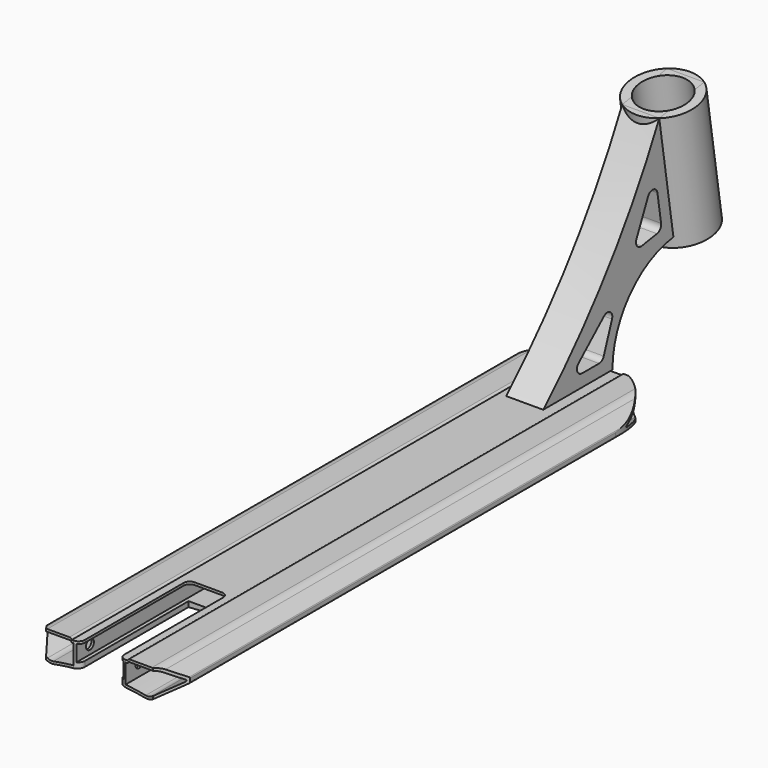
from build123d import *

# Parameters (mm, degrees)
F1_DEPTH       = 250
F2_W           = 38
F2_H           = 13
F3_DEPTH       = 250
F4_T1_DEPTH    = 509.3674969976
F5_R           = 9
F6_R           = 1
F8_DEPTH       = 500.001
F10_DEPTH      = 529
F10_DEPTH_BACK = 27.0742567341
F12_DEPTH      = 27.0742568341
F12_DEPTH_BACK = 530
F13_F1_R       = 4.9999
F13_F2_R       = 5
F13_F3_R       = 5
F13_F4_R       = 4.9999
F13_F5_R       = 5
F15_DEPTH      = 15
F16_R          = 27.5
F17_DEPTH      = 100
F19_D          = 40
F21_D          = 8
F21_DEPTH      = 66
F21_TIP        = 2.4034424761
F23_DEPTH      = 72.5010001
F24_R          = 5


# Not quite as in the source:
# - a fillet or chamfer that OpenCascade refuses, or shapes differently, is made with other operations: its cross-section is extruded or revolved along the edge and cut away or added
# - a fillet or chamfer is up to 0.001 mm smaller than in the source, because OpenCascade refuses the exact size
# - an extrude ends at something that could not be found from the text; its depth is read off the source's solid


with BuildPart() as f1:
    # F0 (on Front) → F1 (new body, symmetric)
    with BuildSketch(Plane.XZ):
        with BuildLine():
            Line((22.5, 25.7732567341), (0, 25.7732567341))
            Line((0, 25.7732567341), (-22.5, 25.7732567341))
            Line((-22.5, 25.7732567341), (-22.5, 27.0732567341))
            Line((-22.5, 27.0732567341), (-45.5824640741, 27.0732567341))
            Line((-45.5824640741, 27.0732567341), (-57.5, 17.0732567341))
            Line((-57.5, 17.0732567341), (-57.5, 13.0732567341))
            Line((-57.5, 13.0732567341), (-40.1794919243, 3.0732567341))
            ThreePointArc((-40.1794919243, 3.0732567341), (0, 7.1508015925), (40.1794919243, 3.0732567341))
            Line((40.1794919243, 3.0732567341), (57.5, 13.0732567341))
            Line((57.5, 13.0732567341), (57.5, 17.0732567341))
            Line((57.5, 17.0732567341), (45.5824640741, 27.0732567341))
            Line((45.5824640741, 27.0732567341), (22.5, 27.0732567341))
            Line((22.5, 27.0732567341), (22.5, 25.7732567341))
        make_face()
    extrude(amount=F1_DEPTH, both=True)

    # F2 (on Front) → F3 (cut, symmetric)
    with BuildSketch(Plane.XZ):
        with Locations((0, 17.2732567341)):
            Rectangle(F2_W, F2_H)
    extrude(amount=F3_DEPTH, both=True, mode=Mode.SUBTRACT)

    # F4: fillet of radius 2 on 2 edges, made by hand

    # F4_s2 → F4_t1 (cut)
    with BuildSketch(Plane.XZ.offset(-254.6837484988)):
        with BuildLine():
            ThreePointArc((-24.3734993995, 27.0732567341), (-23.2333239744, 26.7164244066), (-22.5, 25.7732567341))
            Line((-22.5, 25.7732567341), (-22.5, 27.0732567341))
            Line((-22.5, 27.0732567341), (-24.3734993995, 27.0732567341))
        make_face()
        with BuildLine():
            ThreePointArc((24.3734993995, 27.0732567341), (23.2333239744, 26.7164244066), (22.5, 25.7732567341))
            Line((22.5, 25.7732567341), (22.5, 27.0732567341))
            Line((22.5, 27.0732567341), (24.3734993995, 27.0732567341))
        make_face()
    extrude(amount=F4_T1_DEPTH, mode=Mode.SUBTRACT)

    # F5
    f5_edges = [f1.edges().sort_by_distance(p)[0] for p in [
        (-45.582464, 0, 27.073257),
        (45.582464, 0, 27.073257),
        (40.179492, 0, 3.073257),
        (-40.179492, 0, 3.073257),
    ]]
    fillet(f5_edges, radius=F5_R)

    # F6
    f6_edges = [f1.edges().sort_by_distance(p)[0] for p in [
        (57.5, 0, 17.073257),
        (57.5, 0, 13.073257),
        (-57.5, 0, 17.073257),
        (-57.5, 0, 13.073257),
    ]]
    fillet(f6_edges, radius=F6_R)

    # F7 (on face) → F8 (cut, through all)
    with BuildSketch(Plane.XZ.offset(250)):
        with BuildLine():
            ThreePointArc((-37.3093701274, 5.6753867217), (-29.1789785809, 7.0322344696), (-21, 8.0562519915))
            Line((-21, 8.0562519915), (-21, 10.7732567341))
            Line((-21, 10.7732567341), (-21, 23.7732567341))
            Line((-21, 23.7732567341), (-22.5, 23.7732567341))
            ThreePointArc((-22.5, 23.7732567341), (-23.2333239744, 24.7164244066), (-24.3734993995, 25.0732567341))
            Line((-24.3734993995, 25.0732567341), (-42.3067319657, 25.0732567341))
            ThreePointArc((-42.3067319657, 25.0732567341), (-44.7008729689, 24.6511050796), (-46.8062452335, 23.435567836))
            Line((-46.8062452335, 23.435567836), (-55.7563117574, 15.9255703167))
            ThreePointArc((-55.7563117574, 15.9255703167), (-56.1097188459, 15.0723701308), (-55.6135241478, 14.2935004698))
            Line((-55.6135241478, 14.2935004698), (-42.1022690923, 6.4927737264))
            ThreePointArc((-42.1022690923, 6.4927737264), (-39.7790673433, 5.6545786734), (-37.3093701274, 5.6753867217))
        make_face()
        with BuildLine():
            Line((42.3067319657, 25.0732567341), (24.3734993995, 25.0732567341))
            ThreePointArc((24.3734993995, 25.0732567341), (23.2333239744, 24.7164244066), (22.5, 23.7732567341))
            Line((22.5, 23.7732567341), (21, 23.7732567341))
            Line((21, 23.7732567341), (21, 10.7732567341))
            Line((21, 10.7732567341), (21, 8.0562519915))
            ThreePointArc((21, 8.0562519915), (29.1789785809, 7.0322344696), (37.3093701274, 5.6753867217))
            ThreePointArc((37.3093701274, 5.6753867217), (39.7790673433, 5.6545786734), (42.1022690923, 6.4927737264))
            Line((42.1022690923, 6.4927737264), (55.6135241478, 14.2935004698))
            ThreePointArc((55.6135241478, 14.2935004698), (56.1097188459, 15.0723701308), (55.7563117574, 15.9255703167))
            Line((55.7563117574, 15.9255703167), (46.8062452335, 23.435567836))
            ThreePointArc((46.8062452335, 23.435567836), (44.7008729689, 24.6511050796), (42.3067319657, 25.0732567341))
        make_face()
    extrude(amount=-F8_DEPTH, mode=Mode.SUBTRACT)

    # F9 (on Top) → F10 (cut, two sides)
    with BuildSketch(Plane.XY) as f10_sk:
        with BuildLine():
            ThreePointArc((-57.5, 200), (0, 257.5), (57.5, 200))
            Line((57.5, 200), (57.5, 280))
            Line((57.5, 280), (-57.5, 280))
            Line((-57.5, 280), (-57.5, 200))
        make_face()
    extrude(amount=-F10_DEPTH, mode=Mode.SUBTRACT)
    extrude(f10_sk.sketch, amount=F10_DEPTH_BACK, mode=Mode.SUBTRACT)

    # F11 (on Top) → F12 (cut, two sides)
    with BuildSketch(Plane.XY) as f12_sk:
        Polygon((-43.2975540478, -250), (-68, -216), (-68, -346), (68, -346), (68, -216), (43.2975540478, -250), (16, -250), (16, -140), (-16, -140), (-16, -250), align=None)
    extrude(amount=F12_DEPTH, mode=Mode.SUBTRACT)
    extrude(f12_sk.sketch, amount=-F12_DEPTH_BACK, mode=Mode.SUBTRACT)

    # F13: fillet of radius 5 on 7 edges, made by hand

    # F13_f1 (radius 5 in the source; OpenCascade refuses exactly that, so slightly less here)
    f13_f1_edges = [f1.edges().sort_by_distance(p)[0] for p in [
        (16, -250, 8.6415155184),
    ]]
    fillet(f13_f1_edges, radius=F13_F1_R)

    # F13_f2
    f13_f2_edges = [f1.edges().sort_by_distance(p)[0] for p in [
        (16, -140, 8.6415155184),
    ]]
    fillet(f13_f2_edges, radius=F13_F2_R)

    # F13_f3
    f13_f3_edges = [f1.edges().sort_by_distance(p)[0] for p in [
        (16, -140, 24.7732567341),
    ]]
    fillet(f13_f3_edges, radius=F13_F3_R)

    # F13_f4 (radius 5 in the source; OpenCascade refuses exactly that, so slightly less here)
    f13_f4_edges = [f1.edges().sort_by_distance(p)[0] for p in [
        (-16, -250, 24.7732567341),
    ]]
    fillet(f13_f4_edges, radius=F13_F4_R)

    # F13_f5
    f13_f5_edges = [f1.edges().sort_by_distance(p)[0] for p in [
        (-16, -140, 24.7732567341),
    ]]
    fillet(f13_f5_edges, radius=F13_F5_R)

    # F21 (one way)
    with BuildSketch(Plane.YZ.offset(21)):
        with Locations((-236, 18.0562519915)):
            Circle(F21_D / 2)
    extrude(amount=-F21_DEPTH, mode=Mode.SUBTRACT)
    with Locations(Plane.YZ.offset(21)):
        with Locations((-236, 18.0562519915)):
            with Locations((0, 0, -(F21_DEPTH + F21_TIP / 2))):  # 118° drill point
                Cone(0, F21_D / 2, F21_TIP, mode=Mode.SUBTRACT)


with BuildPart() as f15:
    # F14 (on Right) → F15 (new body, symmetric)
    with BuildSketch(Plane.YZ):
        with BuildLine():
            Line((180, 27.0732567341), (250, 27.0732567341))
            ThreePointArc((250, 27.0732567341), (267.6550746197, 73.5491514208), (311.7145367693, 96.5811778586))
            Line((311.7145367693, 96.5811778586), (313.0254460068, 88.3044226746))
            Line((313.0254460068, 88.3044226746), (358.4591096742, 95.5004080665))
            Line((358.4591096742, 95.5004080665), (342.8156631702, 194.269242126))
            Line((342.8156631702, 194.269242126), (297.3819995028, 187.0732567341))
            ThreePointArc((297.3819995028, 187.0732567341), (245.9666940414, 101.7355345871), (180, 27.0732567341))
        make_face()
    extrude(amount=F15_DEPTH, both=True)

    # F16 (on face) → F17 (join, through all)
    with BuildSketch(Plane(origin=(0, -21.6269522386, 136.547202454), x_dir=(1, 0, 0), z_dir=(0, -0.156434465, 0.9876883406))):
        with Locations((0, 345.9854384523)):
            Circle(F16_R)
    extrude(amount=-F17_DEPTH)

    # F19 (through all)
    with Locations(Plane(origin=(0, -21.6269522386, 136.547202454), x_dir=(1, 0, 0), z_dir=(0, -0.156434465, 0.9876883406))):
        with Locations((0, 345.9854384523)):
            Hole(F19_D / 2)

    # F22 (on face) → F23 (cut, through all)
    with BuildSketch(Plane.YZ.offset(15)):
        Polygon((256.378660542, 82.0732567341), (206, 37.0732567341), (240, 37.0732567341), align=None)
        Polygon((292.9320627918, 150.9321765961), (270.3409635007, 101.7931673181), (299.9716137186, 106.4862012693), align=None)
    extrude(amount=-F23_DEPTH, mode=Mode.SUBTRACT)

    # F24
    f24_edges = [f15.edges().sort_by_distance(p)[0] for p in [
        (0, 292.932063, 150.932177),
        (0, 270.340964, 101.793167),
        (0, 299.971614, 106.486201),
        (0, 240, 37.073257),
        (0, 256.378661, 82.073257),
        (0, 206, 37.073257),
    ]]
    fillet(f24_edges, radius=F24_R)


solid = Compound([f1.part, f15.part])
